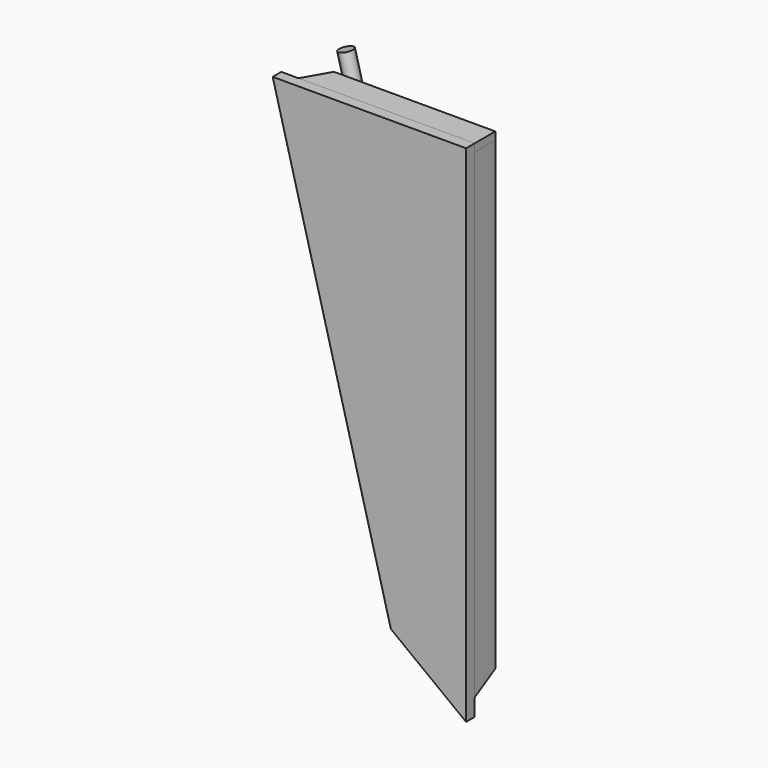
from build123d import *

# Parameters (mm, degrees)
F1_DEPTH  = 25
F2_R      = 16.5
F3_DEPTH  = 100
F6_R      = 16.5
F7_DEPTH  = 982.4856519699
F8_DEPTH  = 80
F9_DEPTH  = 80
F11_DEPTH = 18
F13_DEPTH = 18


with BuildPart() as f1:
    # F0 (on Front) → F1 (new body)
    with BuildSketch(Plane.XZ):
        Polygon((-175, 133.3229162597), (0, 0), (0, 1175), (-450, 1175), align=None)
    extrude(amount=F1_DEPTH)

    # F2 (on face) → F3 (join)
    with BuildSketch(Plane(origin=(0, 0, 0), x_dir=(-1, 0, 0), z_dir=(0, 1, 0))):
        with Locations((372.1045335043, 1115)):
            Circle(F2_R)
        with Locations((122.2474566279, 168.5622138455)):
            Circle(F2_R)
    extrude(amount=F3_DEPTH)


with BuildPart() as f7:
    # F6 (on line) → F7 (new body)
    with BuildSketch(Plane(origin=(-299.4225953601, 0, 1134.1878397842), x_dir=(0.9668744791, 0, 0.2552523099), z_dir=(0.2552523099, 0, -0.9668744791))):
        with Locations((-75.1720515084, -116.5)):
            Circle(F6_R)
    extrude(amount=F7_DEPTH)


with BuildPart() as f8:
    # F8 (new): a face of the model
    f8_faces = [f7.part.faces().sort_by_distance(p)[0] for p in [
        (-372.1045335043, 116.5, 1115),
    ]]
    extrude(f8_faces, amount=F8_DEPTH)


with BuildPart() as f9:
    # F9 (new): a face of the model
    f9_faces = [f7.part.faces().sort_by_distance(p)[0] for p in [
        (-121.322801438, 116.5, 165.0596970396),
    ]]
    extrude(f9_faces, amount=F9_DEPTH)


with BuildPart() as f11:
    # F10 (on face) → F11 (new body)
    with BuildSketch(Plane.XY.offset(1175)):
        Polygon((-410, 0), (0, 0), (0, 60), (-375.3589838486, 60), align=None)
    extrude(amount=-F11_DEPTH)


with BuildPart() as f13:
    # F12 (on face) → F13 (new body)
    with BuildSketch(Plane.YZ):
        Polygon((60, 1157), (0, 1157), (0, 40), (60, 74.6410161514), align=None)
    extrude(amount=-F13_DEPTH)


solid = Compound([f1.part, f7.part, f8.part, f9.part, f11.part, f13.part])
